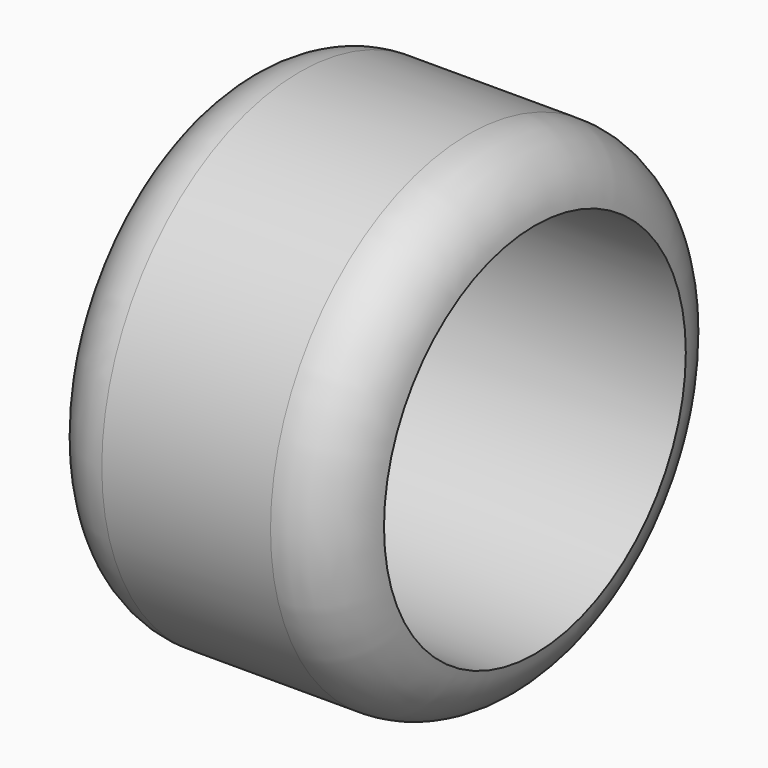
from build123d import *

# Parameters (mm, degrees)
F0_R     = 14.75
F0_R_2   = 11.25
F1_DEPTH = 18


# Not quite as in the source:
# - a fillet or chamfer that OpenCascade refuses, or shapes differently, is made with other operations: its cross-section is extruded or revolved along the edge and cut away or added


with BuildPart() as f1:
    # F0 (on Right) → F1 (new body)
    with BuildSketch(Plane.YZ):
        Circle(F0_R)
        Circle(F0_R_2, mode=Mode.SUBTRACT)
    extrude(amount=F1_DEPTH)

    # F2: fillet of radius 4 on 2 edges, made by hand

    # F2_s1 → F2_t2 (revolve, cut)
    with BuildSketch(Plane.XY):
        with BuildLine():
            ThreePointArc((14.0313730334, 14.75), (16.6771243445, 13.75), (18, 11.25))
            Line((18, 11.25), (18, 14.75))
            Line((18, 14.75), (14.0313730334, 14.75))
        make_face()
    revolve(axis=Axis((18, 0, 0), (1, 0, 0)), mode=Mode.SUBTRACT)

    # F2_s3 → F2_t4 (revolve, cut)
    with BuildSketch(Plane.XY):
        with BuildLine():
            ThreePointArc((3.9686269666, 14.75), (1.3228756555, 13.75), (0, 11.25))
            Line((0, 11.25), (0, 14.75))
            Line((0, 14.75), (3.9686269666, 14.75))
        make_face()
    revolve(axis=Axis((0, 0, 0), (1, 0, 0)), mode=Mode.SUBTRACT)


solid = f1.part
